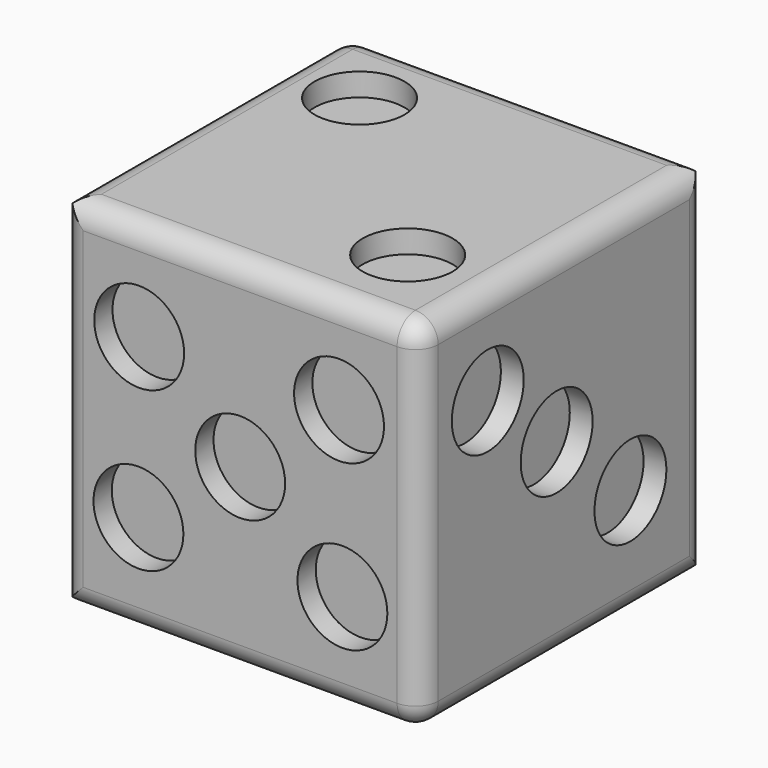
from build123d import *

# Parameters (mm, degrees)
F0_W         = 200
F0_H         = 200
F1_DEPTH     = 200
F2_R         = 12.7
F3_T1_DEPTH  = 206.35
F3_T3_DEPTH  = 174.6
F3_T5_DEPTH  = 206.35
F3_S9_W      = 12.954
F3_S9_H      = 12.954
F3_T10_DEPTH = 12.954
F3_S15_W     = 12.954
F3_S15_H     = 12.954
F3_T16_DEPTH = 12.954
F4_R         = 25
F5_DEPTH     = 12.7
F6_R         = 25
F7_DEPTH     = 12.7
F8_DEPTH     = 12.7
F9_R         = 25
F10_DEPTH    = 12.7
F11_R        = 25
F12_DEPTH    = 12.7
F13_R        = 25
F14_DEPTH    = 12.7
F15_R        = 25
F16_DEPTH    = 12.7


# Not quite as in the source:
# - a fillet or chamfer that OpenCascade refuses, or shapes differently, is made with other operations: its cross-section is extruded or revolved along the edge and cut away or added


with BuildPart() as f1:
    # F0 (on Front) → F1 (new body)
    with BuildSketch(Plane.XZ):
        Rectangle(F0_W, F0_H)
    extrude(amount=F1_DEPTH)

    # F2
    f2_edges = [f1.edges().sort_by_distance(p)[0] for p in [
        (100, -100, -100),
        (100, -100, 100),
        (100, 0, 0),
        (100, -200, 0),
        (0, -200, -100),
        (0, -200, 100),
        (-100, -200, 0),
    ]]
    fillet(f2_edges, radius=F2_R)

    # F3: fillet of radius 12.7 on 11 edges, made by hand

    # F3_s2 → F3_t1 (cut)
    with BuildSketch(Plane.XZ.offset(12.7)):
        with BuildLine():
            ThreePointArc((-100, 87.3), (-96.2802561211, 96.2802561211), (-87.3, 100))
            Line((-87.3, 100), (-100, 100))
            Line((-100, 100), (-100, 87.3))
        make_face()
        with BuildLine():
            ThreePointArc((-87.3, -100), (-96.2802561211, -96.2802561211), (-100, -87.3))
            Line((-100, -87.3), (-100, -100))
            Line((-100, -100), (-87.3, -100))
        make_face()
    extrude(amount=F3_T1_DEPTH, mode=Mode.SUBTRACT)

    # F3_s4 → F3_t3 (cut)
    with BuildSketch(Plane.XY.offset(-87.3)):
        with BuildLine():
            ThreePointArc((-100, -12.7), (-96.2802561211, -3.7197438789), (-87.3, 0))
            Line((-87.3, 0), (-100, 0))
            Line((-100, 0), (-100, -12.7))
        make_face()
    extrude(amount=F3_T3_DEPTH, mode=Mode.SUBTRACT)

    # F3_s6 → F3_t5 (cut)
    with BuildSketch(Plane.YZ.offset(-87.3)):
        with BuildLine():
            ThreePointArc((0, 87.3), (-3.7197438789, 96.2802561211), (-12.7, 100))
            Line((-12.7, 100), (0, 100))
            Line((0, 100), (0, 87.3))
        make_face()
        with BuildLine():
            ThreePointArc((-12.7, -100), (-3.7197438789, -96.2802561211), (0, -87.3))
            Line((0, -87.3), (0, -100))
            Line((0, -100), (-12.7, -100))
        make_face()
    extrude(amount=F3_T5_DEPTH, mode=Mode.SUBTRACT)


with BuildPart() as f3_tool8:
    # F3_s9 → F3_t10 (new body)
    with BuildSketch(Plane.YZ.offset(-87.3)):
        with Locations((-6.223, 93.777)):
            Rectangle(F3_S9_W, F3_S9_H)
    extrude(amount=-F3_T10_DEPTH)

    # F3_s11 → F3_t12 (revolve, cut)
    with BuildSketch(Plane(origin=(-87.3, -12.7, 87.3), x_dir=(0, -0.7071067812, -0.7071067812), z_dir=(0, 0.7071067812, -0.7071067812))):
        with BuildLine():
            ThreePointArc((0, -12.7), (12.7, 0), (0, 12.7))
            Line((0, 12.7), (0, -12.7))
        make_face()
    revolve(axis=Axis((-87.3, -12.7, 87.3), (-1, 0, 0)), mode=Mode.SUBTRACT)


with BuildPart() as f1_1:
    add(f1.part)

    # F3_t7: cut F3_tool8
    add(f3_tool8.part, mode=Mode.SUBTRACT)


with BuildPart() as f3_tool14:
    # F3_s15 → F3_t16 (new body)
    with BuildSketch(Plane.XY.offset(-87.3)):
        with Locations((-93.777, -6.223)):
            Rectangle(F3_S15_W, F3_S15_H)
    extrude(amount=-F3_T16_DEPTH)

    # F3_s17 → F3_t18 (revolve, cut)
    with BuildSketch(Plane(origin=(-87.3, -12.7, -87.3), x_dir=(0.7071067812, -0.7071067812, 0), z_dir=(0.7071067812, 0.7071067812, 0))):
        with BuildLine():
            ThreePointArc((0, -12.7), (12.7, 0), (0, 12.7))
            Line((0, 12.7), (0, -12.7))
        make_face()
    revolve(axis=Axis((-87.3, -12.7, -87.3), (0, 0, -1)), mode=Mode.SUBTRACT)


with BuildPart() as f1_2:
    add(f1_1.part)

    # F3_t13: cut F3_tool14
    add(f3_tool14.part, mode=Mode.SUBTRACT)

    # F4 (on face) → F5 (cut)
    with BuildSketch(Plane(origin=(0, 0, 0), x_dir=(-1, 0, 0), z_dir=(0, 1, 0))):
        Circle(F4_R)
    extrude(amount=-F5_DEPTH, mode=Mode.SUBTRACT)

    # F6 (on face) → F7 (cut)
    with BuildSketch(Plane.XY.offset(100)):
        with Locations((-56.3085600734, -46.6261841357)):
            Circle(F6_R)
        with Locations((52.2117828626, -148.8133593049)):
            Circle(F6_R)
    extrude(amount=-F7_DEPTH, mode=Mode.SUBTRACT)

    # F6 (on face) → F8 (cut)
    with BuildSketch(Plane.XY.offset(100)):
        with Locations((-56.3085600734, -46.6261841357)):
            Circle(F6_R)
        with Locations((52.2117828626, -148.8133593049)):
            Circle(F6_R)
    extrude(amount=-F8_DEPTH, mode=Mode.SUBTRACT)

    # F9 (on face) → F10 (cut)
    with BuildSketch(Plane.YZ.offset(100)):
        with Locations((-152.8625637293, 45.855615288)):
            Circle(F9_R)
        with Locations((-104.9481332302, 6.1764707789)):
            Circle(F9_R)
        with Locations((-53.6647066474, -38.3689813316)):
            Circle(F9_R)
    extrude(amount=-F10_DEPTH, mode=Mode.SUBTRACT)

    # F11 (on face) → F12 (cut)
    with BuildSketch(Plane(origin=(-100, 0, 0), x_dir=(0, -1, 0), z_dir=(-1, 0, 0))):
        with Locations((50.6975390017, -48.2849427062)):
            Circle(F11_R)
        with Locations((48.2081025839, 42.5794422626)):
            Circle(F11_R)
        with Locations((144.8811888695, 41.3347259164)):
            Circle(F11_R)
        with Locations((148.2004225254, -47.8700399399)):
            Circle(F11_R)
    extrude(amount=-F12_DEPTH, mode=Mode.SUBTRACT)

    # F13 (on face) → F14 (cut)
    with BuildSketch(Plane.XZ.offset(200)):
        with Locations((-56.1834387481, 45.481286943)):
            Circle(F13_R)
        with Locations((-56.5915383924, -43.1586373624)):
            Circle(F13_R)
        with Locations((56.8646900356, -45.1069548726)):
            Circle(F13_R)
        with Locations((54.9930334091, 45.8556227386)):
            Circle(F13_R)
        Circle(F13_R)
    extrude(amount=-F14_DEPTH, mode=Mode.SUBTRACT)

    # F15 (on face) → F16 (cut)
    with BuildSketch(Plane(origin=(0, 0, -100), x_dir=(1, 0, 0), z_dir=(0, 0, -1))):
        with Locations((-53.2460398972, 155.2098095417)):
            Circle(F15_R)
        with Locations((-53.4454273642, 99.2308959943)):
            Circle(F15_R)
        with Locations((-54.8167897346, 40.5999273626)):
            Circle(F15_R)
        with Locations((39.449018472, 157.1737299708)):
            Circle(F15_R)
        with Locations((40.3425594879, 98.5919412215)):
            Circle(F15_R)
        with Locations((42.359188109, 39.4558809987)):
            Circle(F15_R)
    extrude(amount=-F16_DEPTH, mode=Mode.SUBTRACT)


solid = f1_2.part
